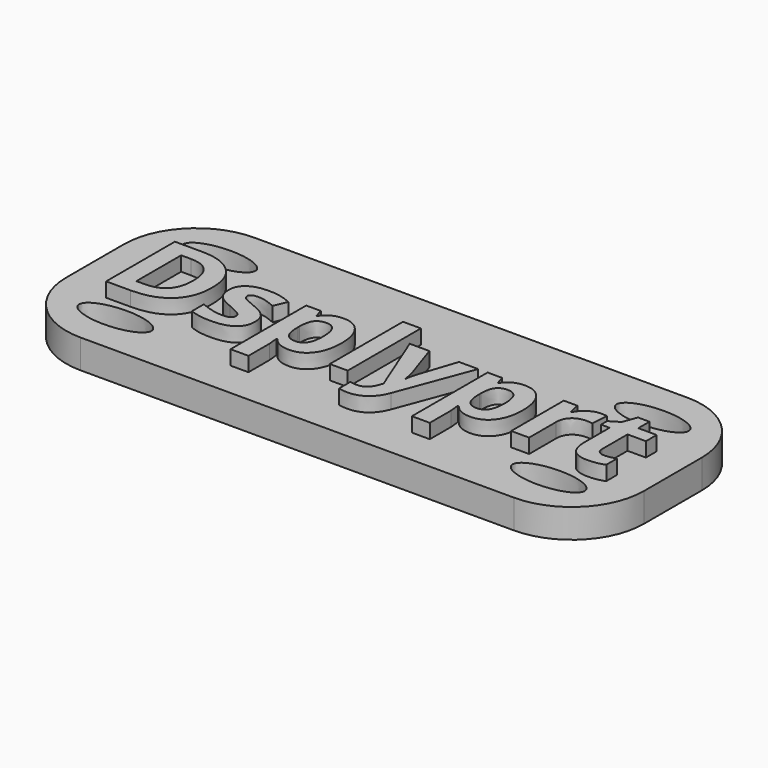
from build123d import *

# Parameters (mm, degrees)
F0_W         = 40
F0_H         = 15
F1_DEPTH     = 2
F2_TEXT_SIZE = 8.3333333333
F3_DEPTH     = 1
F4_R         = 5


# Not quite as in the source:
# - Text() gives the source's letters only with a copy of the font that has no kerning and outlines rounded to 1/6400 em; it was checked with that copy


with BuildPart() as f1:
    # F0 (on Top) → F1 (new body)
    with BuildSketch(Plane.XY):
        Rectangle(F0_W, F0_H)
        with BuildLine():
            add(Edge.make_bspline(
                [(-12.5, -4.5), (-12.5, -2.7679491924), (-16.25, -3.6339745962), (-20, -4.5), (-16.25, -5.3660254038), (-12.5, -6.2320508076), (-12.5, -4.5)],
                knots=[0, 0, 0, 2.0943951024, 2.0943951024, 4.1887902048, 4.1887902048, 6.2831853072, 6.2831853072, 6.2831853072], degree=2, weights=[1, 0.5, 1, 0.5, 1, 0.5, 1]))
        make_face(mode=Mode.SUBTRACT)
        with BuildLine():
            add(Edge.make_bspline(
                [(17.5, -4.5), (17.5, -2.7679491924), (13.75, -3.6339745962), (10, -4.5), (13.75, -5.3660254038), (17.5, -6.2320508076), (17.5, -4.5)],
                knots=[0, 0, 0, 2.0943951024, 2.0943951024, 4.1887902048, 4.1887902048, 6.2831853072, 6.2831853072, 6.2831853072], degree=2, weights=[1, 0.5, 1, 0.5, 1, 0.5, 1]))
        make_face(mode=Mode.SUBTRACT)
        with BuildLine():
            add(Edge.make_bspline(
                [(-12.5, 4.5), (-12.5, 6.2320508076), (-16.25, 5.3660254038), (-20, 4.5), (-16.25, 3.6339745962), (-12.5, 2.7679491924), (-12.5, 4.5)],
                knots=[0, 0, 0, 2.0943951024, 2.0943951024, 4.1887902048, 4.1887902048, 6.2831853072, 6.2831853072, 6.2831853072], degree=2, weights=[1, 0.5, 1, 0.5, 1, 0.5, 1]))
        make_face(mode=Mode.SUBTRACT)
        with BuildLine():
            add(Edge.make_bspline(
                [(17.5, 4.5), (17.5, 6.2320508076), (13.75, 5.3660254038), (10, 4.5), (13.75, 3.6339745962), (17.5, 2.7679491924), (17.5, 4.5)],
                knots=[0, 0, 0, 2.0943951024, 2.0943951024, 4.1887902048, 4.1887902048, 6.2831853072, 6.2831853072, 6.2831853072], degree=2, weights=[1, 0.5, 1, 0.5, 1, 0.5, 1]))
        make_face(mode=Mode.SUBTRACT)
    extrude(amount=F1_DEPTH)

    # F4
    f4_edges = [f1.edges().sort_by_distance(p)[0] for p in [
        (-20, -7.5, 1),
        (20, -7.5, 1),
        (20, 7.5, 1),
        (-20, 7.5, 1),
    ]]
    fillet(f4_edges, radius=F4_R)


with BuildPart() as f3:
    # F2 (on face) → F3 (new body)
    with BuildSketch(Plane.XY.offset(2)):
        with Locations((-17.5868192361, -3)):
            Text('Dsplyprt', F2_TEXT_SIZE, font='Open Sans', font_style=FontStyle.BOLD, text_align=(TextAlign.LEFT, TextAlign.BOTTOM))
    extrude(amount=F3_DEPTH)


solid = Compound([f1.part, f3.part])
